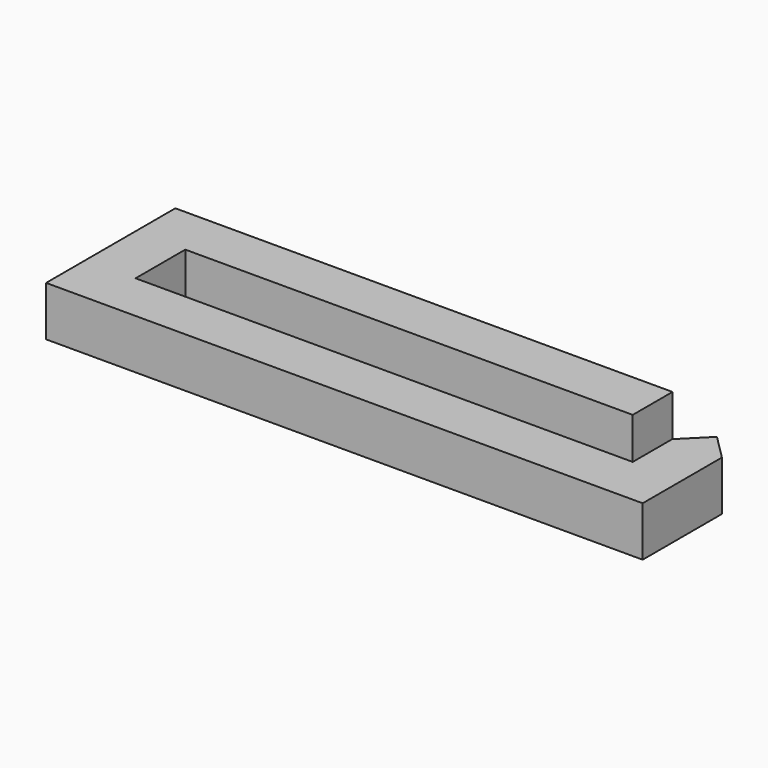
from build123d import *

# Parameters (mm, degrees)
F0_W     = 4
F0_H     = 5
F0_H_2   = 5.9711672319
F1_DEPTH = 4
F2_SIZE  = 1.99999


# Not quite as in the source:
# - a fillet or chamfer is up to 0.001 mm smaller than in the source, because OpenCascade refuses the exact size


with BuildPart() as f1:
    # F0 (on Top) → F1 (new body)
    with BuildSketch(Plane.XY):
        with Locations((-21, -0.121395904)):
            Rectangle(F0_W, F0_H)
        Polygon((-19, -2.621395904), (-23, -2.621395904), (-23, -6.621395904), (25, -6.621395904), (25, -2.621395904), (21, -2.621395904), align=None)
        Polygon((-23, 6.378604096), (-23, 2.378604096), (-19, 2.378604096), (17, 2.378604096), (17, 6.378604096), align=None)
        with Locations((23, 0.364187712)):
            Rectangle(F0_W, F0_H_2)
    extrude(amount=F1_DEPTH)

    # F2 (size 2 in the source; OpenCascade refuses exactly that, so slightly less here)
    f2_edges = [f1.edges().sort_by_distance(p)[0] for p in [
        (21, 3.349771, 2),
        (25, 3.349771, 2),
    ]]
    chamfer(f2_edges, length=F2_SIZE)


solid = f1.part
